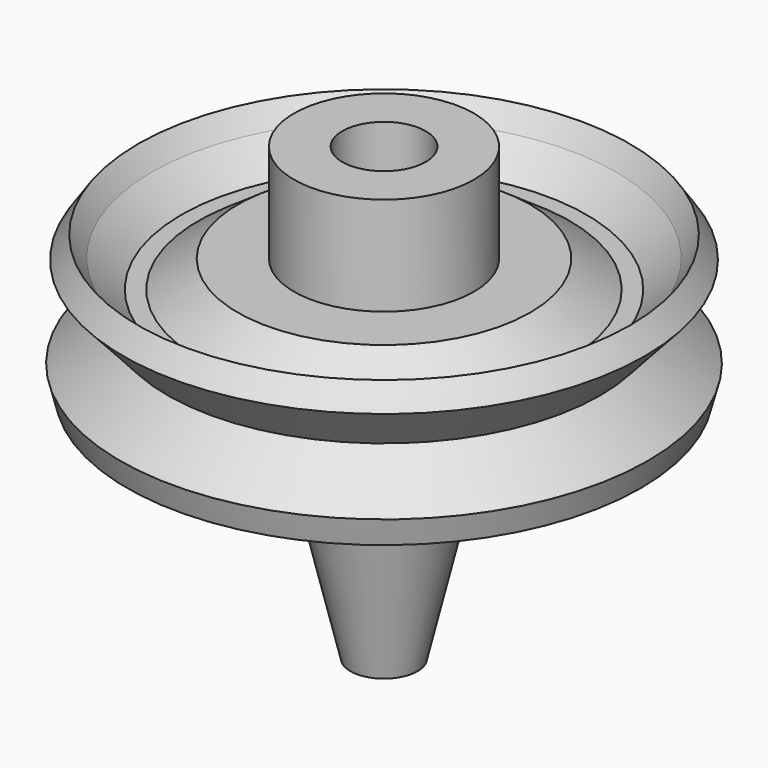
from build123d import *

# Parameters (mm, degrees)
F2_R     = 4.699
F3_DEPTH = 9.398
F4_R     = 1.5367
F5_DEPTH = 17.145


# Not quite as in the source:
# - a feature names something its author has since deleted; it is built from what else it names


with BuildPart() as f1:
    # F0 (on Front) → F1 (revolve)
    with BuildSketch(Plane.XZ):
        Polygon((0, 27.8836265206), (0, -12.487935467), (3.7766563474, -12.487935467), (9.4925444573, 11.6318371147), (16.9307440519, 15.3280049562), (20.9119780944, 19.6802802384), (22.9117851704, 19.6802802384), (27.146894104, 16.1157515753), (28.938142141, 13.8561455533), (29.718, 16.8109368533), (24.366803943, 21.5609171673), (29.371801322, 27.0814523101), (27.6893377921, 29.5746776597), (26.144035833, 27.2886776597), (22.8029862046, 24.1410490125), (20.9119780944, 24.1410490125), (16.4766563474, 27.2050067903), (10.1266563474, 27.2050067903), (10.1266563474, 38.312064533), (0, 38.312064533), align=None)
    revolve(axis=Axis((0, 0, 7.6978455268), (0, 0, -1)))

    # F2 (on face) → F3 (cut)
    with BuildSketch(Plane.XY.offset(38.312064533)):
        Circle(F2_R)
    extrude(amount=-F3_DEPTH, mode=Mode.SUBTRACT)

    # F4 (on face) → F5 (cut)
    with BuildSketch(Plane(origin=(0, 0, -12.487935467), x_dir=(1, 0, 0), z_dir=(0, 0, -1))):
        Circle(F4_R)
    extrude(amount=-F5_DEPTH, mode=Mode.SUBTRACT)


solid = f1.part
